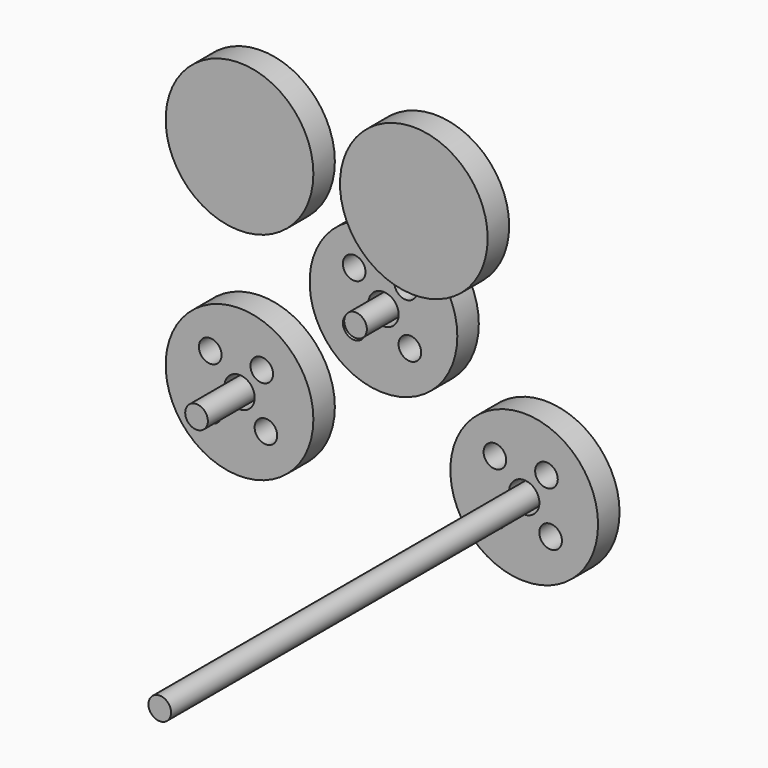
from build123d import *

# Parameters (mm, degrees)
F0_R     = 69.85
F0_R_2   = 10.7048166644
F0_R_3   = 14.3504130315
F2_DEPTH = 25.4
F3_DEPTH = 76.2
F5_DEPTH = 25.4
F9_DEPTH = 381


# Not quite as in the source:
# - the program builds the solid bodies; features that only make, move or delete a surface that nothing else refers to are left out


with BuildPart() as f2:
    # F0 (on Front) → F2 (new body)
    with BuildSketch(Plane.XZ):
        Circle(F0_R)
        with Locations((-27.7036573018, -24.0885839799)):
            Circle(F0_R_2, mode=Mode.SUBTRACT)
        with Locations((24.9833024934, -24.6799281766)):
            Circle(F0_R_2, mode=Mode.SUBTRACT)
        Circle(F0_R_3, mode=Mode.SUBTRACT)
        with Locations((-27.7036573018, 25.2788065644)):
            Circle(F0_R_2, mode=Mode.SUBTRACT)
        with Locations((21.0469203509, 25.2788065644)):
            Circle(F0_R_2, mode=Mode.SUBTRACT)
    extrude(amount=F2_DEPTH)


with BuildPart() as f3:
    # F0 (on Front) → F3 (new body)
    with BuildSketch(Plane.XZ):
        Circle(F0_R_2)
    extrude(amount=F3_DEPTH)


with BuildPart() as f5:
    # F0 (on Front) → F5 (new body)
    with BuildSketch(Plane.XZ):
        with Locations((0, 204.3686956167)):
            Circle(F0_R)
    extrude(amount=F5_DEPTH)


with BuildPart() as f6_1:
    # F6: copy of F2
    add(f2.part.moved(Location((269.24, 0, 0))))


with BuildPart() as f7_1:
    # F7: copy of F3
    add(f3.part.moved(Location((270.002, 0, 0))))

    # F9 (add): a face of the model
    f9_faces = [f7_1.faces().sort_by_distance(p)[0] for p in [
        (270.002, -76.2, 0),
    ]]
    extrude(f9_faces, amount=F9_DEPTH)


with BuildPart() as f8_1:
    # F8: copy of F5
    add(f5.part.moved(Location((164.846, 0, 0))))


with BuildPart() as f10_1:
    # F10: copy of F2
    add(f2.part.moved(Location((0, 170.18, 0))))


with BuildPart() as f11_1:
    # F11: copy of F3
    add(f3.part.moved(Location((0, 187.96, 0))))


solid = Compound([f2.part, f3.part, f5.part, f6_1.part, f7_1.part, f8_1.part, f10_1.part, f11_1.part])
